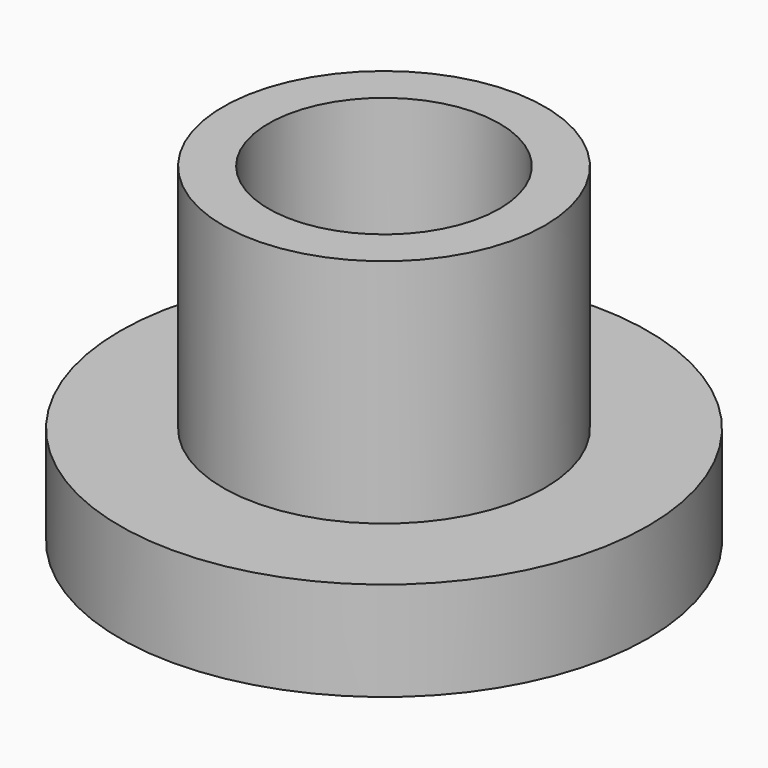
from build123d import *

# Parameters (mm, degrees)
F0_R     = 8
F0_R_2   = 4.875
F1_DEPTH = 3
F0_R_3   = 3.5
F2_DEPTH = 10


# Not quite as in the source:
# - a feature names something its author has since deleted; it is built from what else it names


with BuildPart() as f1:
    # F0 (on Top) → F1 (new body)
    with BuildSketch(Plane.XY):
        with Locations((-9.4900550321, 0)):
            Circle(F0_R)
        with Locations((-9.4900550321, 0)):
            Circle(F0_R_2, mode=Mode.SUBTRACT)
    extrude(amount=F1_DEPTH)


with BuildPart() as f2:
    # F0 (on Top) → F2 (new body)
    with BuildSketch(Plane.XY):
        with Locations((-9.4900550321, 0)):
            Circle(F0_R_2)
        with Locations((-9.4900550321, 0)):
            Circle(F0_R_3, mode=Mode.SUBTRACT)
    extrude(amount=F2_DEPTH)


solid = Compound([f1.part, f2.part])
